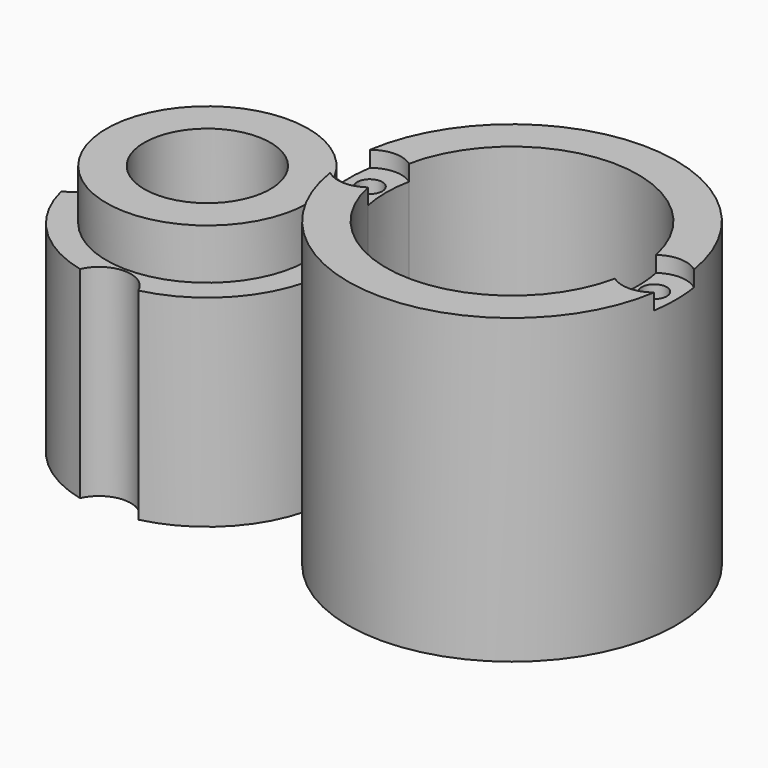
from build123d import *

# Parameters (mm, degrees)
F0_R      = 7.9375
F0_R_2    = 6.35
F1_DEPTH  = 12.7
F3_DEPTH  = 12.701
F4_DEPTH  = 1
F2_R      = 6.35
F5_DEPTH  = 3.175
F7_D      = 7.9375
F8_R      = 10.31875
F8_R_2    = 7.9375
F9_DEPTH  = 19.05
F11_DEPTH = 13.97
F10_R     = 0.7874
F12_DEPTH = 6.35
F13_DEPTH = 1
F14_DEPTH = 10.033


with BuildPart() as f1:
    # F0 (on Top) → F1 (new body)
    with BuildSketch(Plane.XY):
        Circle(F0_R)
        Circle(F0_R_2, mode=Mode.SUBTRACT)
        Circle(F0_R_2)
    extrude(amount=F1_DEPTH)

    # F2 (on face) → F3 (cut, through all)
    with BuildSketch(Plane.XY.offset(12.7)):
        with BuildLine():
            ThreePointArc((1.8335229418, 7.722829784), (0, 7.9375), (-1.8335229418, 7.722829784))
            ThreePointArc((-1.8335229418, 7.722829784), (0, 6.5217), (1.8335229418, 7.722829784))
        make_face()
        with BuildLine():
            ThreePointArc((1.8335229418, -7.722829784), (0, -6.5217), (-1.8335229418, -7.722829784))
            ThreePointArc((-1.8335229418, -7.722829784), (0, -7.9375), (1.8335229418, -7.722829784))
        make_face()
    extrude(amount=-F3_DEPTH, mode=Mode.SUBTRACT)

    # F2 (on face) → F4 (cut)
    with BuildSketch(Plane.XY.offset(12.7)):
        with BuildLine():
            ThreePointArc((-6.5217, 0), (-6.8487175685, 1.0959606672), (-7.722829784, 1.8335229418))
            ThreePointArc((-7.722829784, 1.8335229418), (-7.9375, 0), (-7.722829784, -1.8335229418))
            ThreePointArc((-7.722829784, -1.8335229418), (-6.8487175685, -1.0959606672), (-6.5217, 0))
        make_face()
        with BuildLine():
            ThreePointArc((7.9375, 0), (7.8836497785, 0.9230235208), (7.722829784, 1.8335229418))
            ThreePointArc((7.722829784, 1.8335229418), (6.5217, 0), (7.722829784, -1.8335229418))
            ThreePointArc((7.722829784, -1.8335229418), (7.8836497785, -0.9230235208), (7.9375, 0))
        make_face()
    extrude(amount=-F4_DEPTH, mode=Mode.SUBTRACT)

    # F2 (on face) → F5 (join)
    with BuildSketch(Plane.XY.offset(12.7)):
        Circle(F2_R)
    extrude(amount=F5_DEPTH)

    # F7 (through all)
    with Locations(Plane.XY.offset(15.875)):
        with Locations((0, 0)):
            Hole(F7_D / 2)

    # F0 (on Top) → F14 (cut)
    with BuildSketch(Plane.XY):
        Circle(F0_R_2)
    extrude(amount=F14_DEPTH, mode=Mode.SUBTRACT)


with BuildPart() as f9:
    # F8 (on Top) → F9 (new body)
    with BuildSketch(Plane.XY):
        with Locations((19.1790115059, 0)):
            Circle(F8_R)
        with Locations((19.1790115059, 0)):
            Circle(F8_R_2, mode=Mode.SUBTRACT)
        with Locations((19.1790115059, 0)):
            Circle(F8_R_2)
    extrude(amount=F9_DEPTH)

    # F10 (on face) → F11 (cut)
    with BuildSketch(Plane.XY.offset(19.05)):
        with BuildLine():
            ThreePointArc((26.9507805627, -1.6135402003), (27.0749700652, -0.8110145997), (27.1165115059, 0))
            ThreePointArc((27.1165115059, 0), (27.0749700652, 0.8110145997), (26.9507805627, 1.6135402003))
            ThreePointArc((26.9507805627, 1.6135402003), (19.1790115059, 7.9375), (11.4072424492, 1.6135402003))
            ThreePointArc((11.4072424492, 1.6135402003), (11.2415115059, 0), (11.4072424492, -1.6135402003))
            ThreePointArc((11.4072424492, -1.6135402003), (19.1790115059, -7.9375), (26.9507805627, -1.6135402003))
        make_face()
    extrude(amount=-F11_DEPTH, mode=Mode.SUBTRACT)

    # F10 (on face) → F12 (cut)
    with BuildSketch(Plane.XY.offset(19.05)):
        with Locations((10.2255115059, 0)):
            Circle(F10_R)
        with Locations((28.1325115059, 0)):
            Circle(F10_R)
    extrude(amount=-F12_DEPTH, mode=Mode.SUBTRACT)

    # F10 (on face) → F13 (cut)
    with BuildSketch(Plane.XY.offset(19.05)):
        with BuildLine():
            ThreePointArc((11.4072424492, -1.6135402003), (11.2415115059, 0), (11.4072424492, 1.6135402003))
            ThreePointArc((11.4072424492, 1.6135402003), (10.1850977046, 1.9995916395), (8.97954963, 1.5644740342))
            ThreePointArc((8.97954963, 1.5644740342), (8.8602615059, 0), (8.97954963, -1.5644740342))
            ThreePointArc((8.97954963, -1.5644740342), (10.1850977046, -1.9995916395), (11.4072424492, -1.6135402003))
        make_face()
        with Locations((10.2255115059, 0)):
            Circle(F10_R, mode=Mode.SUBTRACT)
        with BuildLine():
            ThreePointArc((26.9507805627, 1.6135402003), (27.0749700652, 0.8110145997), (27.1165115059, 0))
            ThreePointArc((27.1165115059, 0), (27.0749700652, -0.8110145997), (26.9507805627, -1.6135402003))
            ThreePointArc((26.9507805627, -1.6135402003), (28.1729253073, -1.9995916395), (29.3784733819, -1.5644740342))
            ThreePointArc((29.3784733819, -1.5644740342), (29.4678962559, -0.784507594), (29.4977615059, 0))
            ThreePointArc((29.4977615059, 0), (29.4678962559, 0.784507594), (29.3784733819, 1.5644740342))
            ThreePointArc((29.3784733819, 1.5644740342), (28.1729253073, 1.9995916395), (26.9507805627, 1.6135402003))
        make_face()
        with Locations((28.1325115059, 0)):
            Circle(F10_R, mode=Mode.SUBTRACT)
    extrude(amount=-F13_DEPTH, mode=Mode.SUBTRACT)


solid = Compound([f1.part, f9.part])
